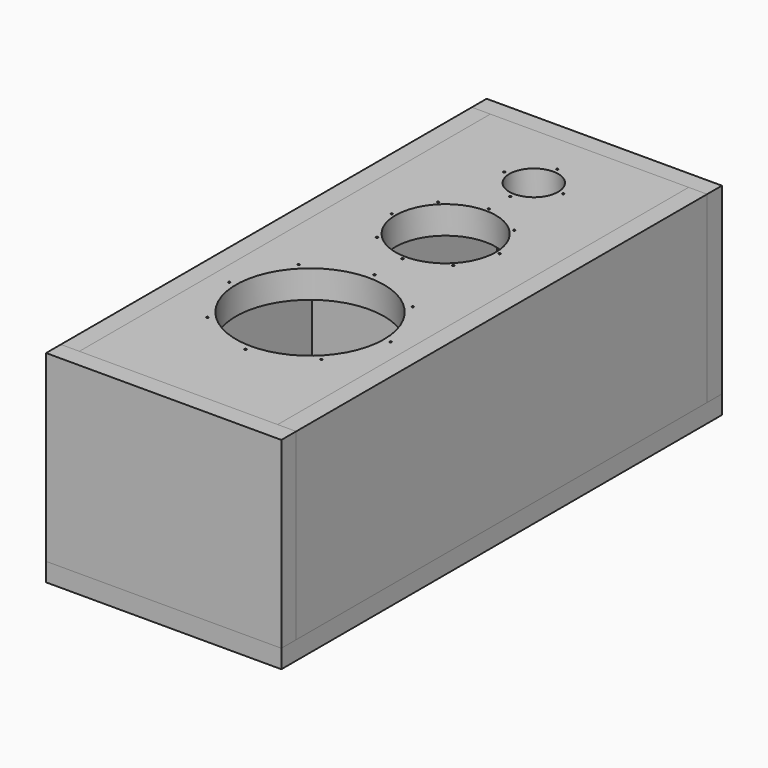
from build123d import *

# Parameters (mm, degrees)
F0_W             = 386
F0_H             = 1000
F1_DEPTH         = 54
F2_R             = 144
F2_R_2           = 97.5
F2_R_3           = 47.5
F3_DEPTH         = 80
F4_W             = 1000
F4_H             = 357
F5_DEPTH         = 36
F6_W             = 1000
F6_H             = 357
F7_DEPTH         = 36
F8_W             = 294
F8_H             = 446
F8_W_2           = 258
F8_H_2           = 410
F9_DEPTH         = 180
F10_W            = 294
F10_H            = 446
F11_DEPTH        = 18
F12_W            = 458
F12_H            = 357
F13_DEPTH        = 36
F14_W            = 458
F14_H            = 357
F15_DEPTH        = 36
F16_W            = 458
F16_H            = 1072
F17_DEPTH        = 36
F19_D            = 4
F19_COPIES_COUNT = 8
F21_D            = 4
F21_COPIES_COUNT = 8
F23_D            = 4
F23_COPIES_COUNT = 4


# Not quite as in the source:
# - a pattern or mirror of a feature is missing from the dataset's text; its kind, count and spacing are read off the source's solid


with BuildPart() as f1:
    # F0 (on Top) → F1 (new body)
    with BuildSketch(Plane.XY):
        Rectangle(F0_W, F0_H)
    extrude(amount=F1_DEPTH)

    # F2 (on face) → F3 (cut)
    with BuildSketch(Plane.XY.offset(54)):
        with Locations((0, -180)):
            Circle(F2_R)
        with Locations((0, 150)):
            Circle(F2_R_2)
        with Locations((0, 364.5142316818)):
            Circle(F2_R_3)
    extrude(amount=-F3_DEPTH, mode=Mode.SUBTRACT)

    # F19 (through all)
    with Locations(Plane.XY.offset(54)):
        with Locations((0, -337)):
            f19 = Hole(F19_D / 2)

    # F19_copies: F19 ×8 about axis
    f19_copies_axis = Axis((0, -180, 0), (0, 0, 1))
    for i in range(1, F19_COPIES_COUNT):
        add(f19.rotate(f19_copies_axis, i * 360 / F19_COPIES_COUNT), mode=Mode.SUBTRACT)

    # F21 (through all)
    with Locations(Plane.XY.offset(54)):
        with Locations((0, 45)):
            f21 = Hole(F21_D / 2)

    # F21_copies: F21 ×8 about axis
    f21_copies_axis = Axis((0, 150, 0), (0, 0, 1))
    for i in range(1, F21_COPIES_COUNT):
        add(f21.rotate(f21_copies_axis, i * 360 / F21_COPIES_COUNT), mode=Mode.SUBTRACT)

    # F23 (through all)
    with Locations(Plane.XY.offset(54)):
        with Locations((0, 307.0142316818)):
            f23 = Hole(F23_D / 2)

    # F23_copies: F23 ×4 about axis
    f23_copies_axis = Axis((0, 364.514232, 0), (0, 0, 1))
    for i in range(1, F23_COPIES_COUNT):
        add(f23.rotate(f23_copies_axis, i * 360 / F23_COPIES_COUNT), mode=Mode.SUBTRACT)


with BuildPart() as f5:
    # F4 (on face) → F5 (new body)
    with BuildSketch(Plane(origin=(-193, 0, 0), x_dir=(0, -1, 0), z_dir=(-1, 0, 0))):
        with Locations((0, -124.5)):
            Rectangle(F4_W, F4_H)
    extrude(amount=F5_DEPTH)


with BuildPart() as f7:
    # F6 (on face) → F7 (new body)
    with BuildSketch(Plane.YZ.offset(193)):
        with Locations((0, -124.5)):
            Rectangle(F6_W, F6_H)
    extrude(amount=F7_DEPTH)


with BuildPart() as f9:
    # F8 (on face) → F9 (new body)
    with BuildSketch(Plane(origin=(0, 0, 0), x_dir=(1, 0, 0), z_dir=(0, 0, -1))):
        with Locations((0, -231)):
            Rectangle(F8_W, F8_H)
        with Locations((0, -231)):
            Rectangle(F8_W_2, F8_H_2, mode=Mode.SUBTRACT)
    extrude(amount=F9_DEPTH)


with BuildPart() as f11:
    # F10 (on face) → F11 (new body)
    with BuildSketch(Plane(origin=(0, 0, -180), x_dir=(1, 0, 0), z_dir=(0, 0, -1))):
        with Locations((0, -231)):
            Rectangle(F10_W, F10_H)
    extrude(amount=F11_DEPTH)


with BuildPart() as f13:
    # F12 (on face) → F13 (new body)
    with BuildSketch(Plane(origin=(0, 500, 0), x_dir=(-1, 0, 0), z_dir=(0, 1, 0))):
        with Locations((0, -124.5)):
            Rectangle(F12_W, F12_H)
    extrude(amount=F13_DEPTH)


with BuildPart() as f15:
    # F14 (on face) → F15 (new body)
    with BuildSketch(Plane.XZ.offset(500)):
        with Locations((0, -124.5)):
            Rectangle(F14_W, F14_H)
    extrude(amount=F15_DEPTH)


with BuildPart() as f17:
    # F16 (on face) → F17 (new body)
    with BuildSketch(Plane(origin=(0, 0, -303), x_dir=(1, 0, 0), z_dir=(0, 0, -1))):
        Rectangle(F16_W, F16_H)
    extrude(amount=F17_DEPTH)


solid = Compound([f1.part, f5.part, f7.part, f9.part, f11.part, f13.part, f15.part, f17.part])
